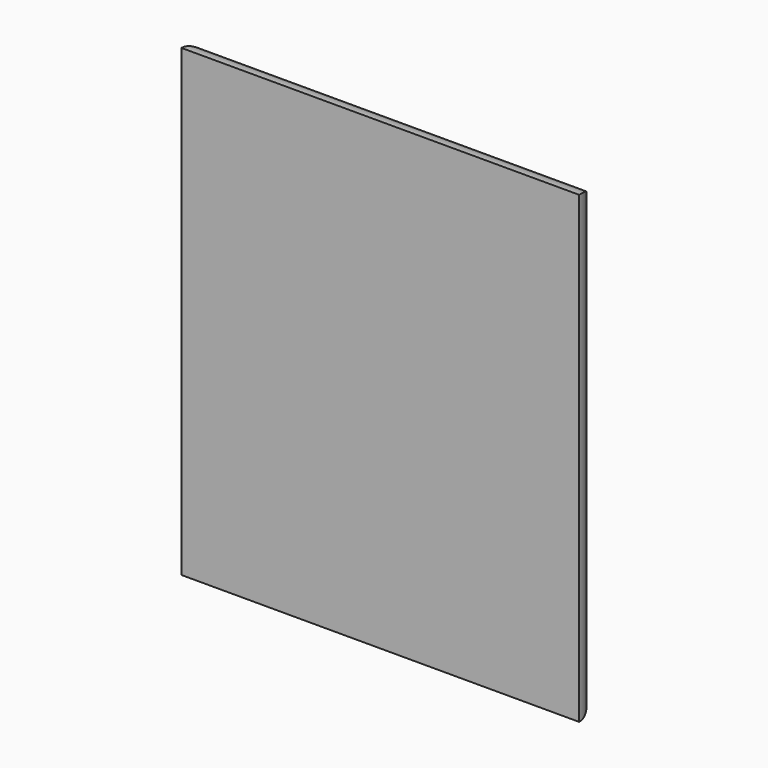
from build123d import *

# Parameters (mm, degrees)
F1_DEPTH = 88.9
F2_DEPTH = 38.1
F3_W     = 3.048
F3_H     = 6.096
F4_DEPTH = 76.201
F5_R     = 5.07999


# Not quite as in the source:
# - a fillet or chamfer is up to 0.001 mm smaller than in the source, because OpenCascade refuses the exact size


with BuildPart() as f1:
    # F0 (on Top) → F1 (new body)
    with BuildSketch(Plane.XY):
        Polygon((-3.5306826939, -16.4269548038), (-16.2306826939, -16.4269548038), (-38.1, -16.4269548038), (-38.1, -21.5069548038), (38.1, -21.5069548038), (38.1, -16.4269548038), (16.2306826939, -16.4269548038), (3.5306826939, -16.4269548038), align=None)
    extrude(amount=F1_DEPTH)

    # F0 (on Top) → F2 (join)
    with BuildSketch(Plane.XY):
        with BuildLine():
            ThreePointArc((14.265, 0), (0, -14.265), (-14.265, 0))
            Line((-14.265, 0), (-16.8021, 0))
            ThreePointArc((-16.8021, 0), (-16.6586331687, -2.1910055589), (-16.2306826939, -4.344594768))
            Line((-16.2306826939, -4.344594768), (-16.2306826939, -16.4269548038))
            Line((-16.2306826939, -16.4269548038), (-3.5306826939, -16.4269548038))
            Line((-3.5306826939, -16.4269548038), (3.5306826939, -16.4269548038))
            Line((3.5306826939, -16.4269548038), (16.2306826939, -16.4269548038))
            Line((16.2306826939, -16.4269548038), (16.2306826939, -4.344594768))
            ThreePointArc((16.2306826939, -4.344594768), (16.6586331687, -2.1910055589), (16.8021, 0))
            Line((16.8021, 0), (14.265, 0))
        make_face()
    extrude(amount=F2_DEPTH)

    # F3 (on face) → F4 (cut, through all)
    with BuildSketch(Plane.YZ.offset(38.1)):
        with Locations((-14.9029548038, 8.7181735593)):
            Rectangle(F3_W, F3_H)
        with Locations((-14.9029548038, 28.7483400475)):
            Rectangle(F3_W, F3_H)
    extrude(amount=-F4_DEPTH, mode=Mode.SUBTRACT)

    # F5 (radius 5.08 in the source; OpenCascade refuses exactly that, so slightly less here)
    f5_edges = [f1.edges().sort_by_distance(p)[0] for p in [
        (0, -16.426955, 88.9),
        (38.1, -16.426955, 44.45),
        (27.165341, -16.426955, 0),
        (-38.1, -16.426955, 44.45),
        (-27.165341, -16.426955, 0),
        (16.230683, -10.385775, 38.1),
        (-16.230683, -10.385775, 38.1),
    ]]
    fillet(f5_edges, radius=F5_R)


solid = f1.part
